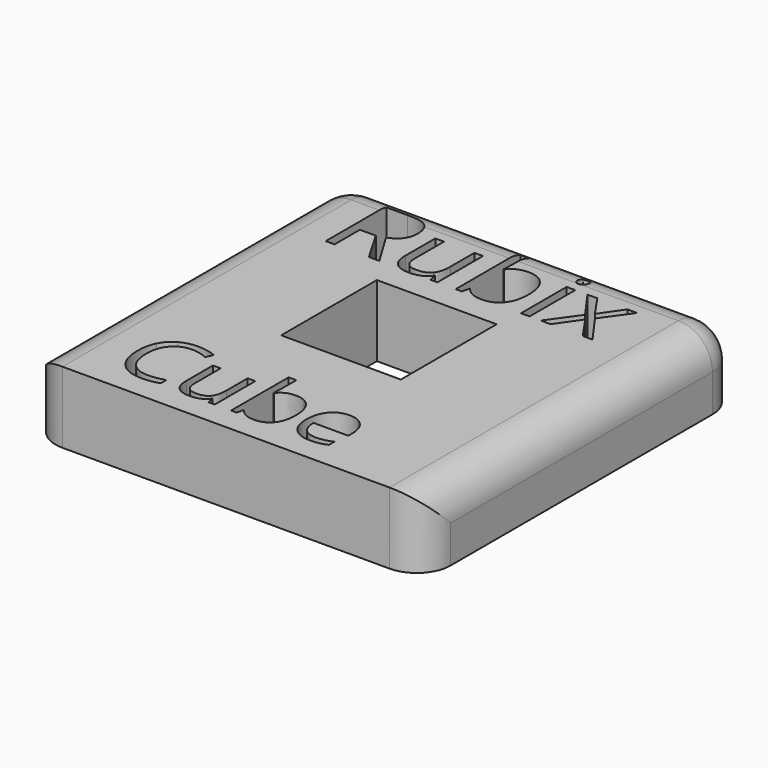
from build123d import *

# Parameters (mm, degrees)
F0_W         = 58.1
F0_H         = 58.1
F0_W_2       = 17.6
F0_H_2       = 17.6
F0_W_3       = 1.2705228995
F0_H_3       = 8.3844719282
F1_DEPTH     = 10.5
F2_T1_DEPTH  = 48.1
F2_T3_DEPTH  = 65.6
F2_T5_DEPTH  = 35.5
F2_T7_DEPTH  = 18
F2_S11_W     = 5
F2_S11_H     = 5
F2_T12_DEPTH = 5
F2_S17_W     = 5
F2_S17_H     = 5
F2_T18_DEPTH = 5


# Not quite as in the source:
# - a fillet or chamfer that OpenCascade refuses, or shapes differently, is made with other operations: its cross-section is extruded or revolved along the edge and cut away or added


with BuildPart() as f1:
    # F0 (on Top) → F1 (new body)
    with BuildSketch(Plane.XY):
        with Locations((-12.3929342572, -6.4361356199)):
            Rectangle(F0_W, F0_H)
        with BuildLine():
            add(Edge.make_bspline(
                [(-25.1530124377, -23.3911235684), (-26.2823661029, -22.8623510431), (-27.411719768, -22.8623510431)],
                knots=[0, 0, 0, 1, 1, 1], degree=2))
            add(Edge.make_bspline(
                [(-27.411719768, -22.8623510431), (-29.0502617908, -22.8623510431), (-29.9990059102, -23.9536243824)],
                knots=[0, 0, 0, 1, 1, 1], degree=2))
            add(Edge.make_bspline(
                [(-29.9990059102, -23.9536243824), (-30.9477500297, -25.0448977216), (-30.9477500297, -26.9423859605)],
                knots=[0, 0, 0, 1, 1, 1], degree=2))
            add(Edge.make_bspline(
                [(-30.9477500297, -26.9423859605), (-30.9477500297, -28.8920986463), (-30.0327341989, -29.957259762)],
                knots=[0, 0, 0, 1, 1, 1], degree=2))
            add(Edge.make_bspline(
                [(-30.0327341989, -29.957259762), (-29.1177183681, -31.0224208778), (-27.4247758797, -31.0224208778)],
                knots=[0, 0, 0, 1, 1, 1], degree=2))
            add(Edge.make_bspline(
                [(-27.4247758797, -31.0224208778), (-26.3846389781, -31.0224208778), (-25.0507395625, -30.6481456747)],
                knots=[0, 0, 0, 1, 1, 1], degree=2))
            Line((-25.0507395625, -30.6481456747), (-25.0507395625, -31.6599943342))
            add(Edge.make_bspline(
                [(-25.0507395625, -31.6599943342), (-26.0843484082, -32.0495016676), (-27.6010333881, -32.0495016676)],
                knots=[0, 0, 0, 1, 1, 1], degree=2))
            add(Edge.make_bspline(
                [(-27.6010333881, -32.0495016676), (-29.7966361783, -32.0495016676), (-30.9901823928, -30.715602252)],
                knots=[0, 0, 0, 1, 1, 1], degree=2))
            add(Edge.make_bspline(
                [(-30.9901823928, -30.715602252), (-32.1837286073, -29.3817028364), (-32.1837286073, -26.9271538301)],
                knots=[0, 0, 0, 1, 1, 1], degree=2))
            add(Edge.make_bspline(
                [(-32.1837286073, -26.9271538301), (-32.1837286073, -25.3908846826), (-31.6092596909, -24.235418794)],
                knots=[0, 0, 0, 1, 1, 1], degree=2))
            add(Edge.make_bspline(
                [(-31.6092596909, -24.235418794), (-31.0347907746, -23.0799529054), (-29.9500454912, -22.4543475514)],
                knots=[0, 0, 0, 1, 1, 1], degree=2))
            add(Edge.make_bspline(
                [(-29.9500454912, -22.4543475514), (-28.8653002079, -21.8287421974), (-27.3964876376, -21.8287421974)],
                knots=[0, 0, 0, 1, 1, 1], degree=2))
            add(Edge.make_bspline(
                [(-27.3964876376, -21.8287421974), (-25.8341062666, -21.8287421974), (-24.6634082477, -22.3988590765)],
                knots=[0, 0, 0, 1, 1, 1], degree=2))
            Line((-24.6634082477, -22.3988590765), (-25.1530124377, -23.3911235684))
        make_face(mode=Mode.SUBTRACT)
        with BuildLine():
            Line((-23.1314911374, -24.4595487121), (-21.9890813605, -24.4595487121))
            Line((-21.9890813605, -24.4595487121), (-21.9890813605, -29.2946620915))
            add(Edge.make_bspline(
                [(-21.9890813605, -29.2946620915), (-21.9890813605, -30.2064138943), (-21.5745498129, -30.6546737306)],
                knots=[0, 0, 0, 1, 1, 1], degree=2))
            add(Edge.make_bspline(
                [(-21.5745498129, -30.6546737306), (-21.1600182653, -31.1029335668), (-20.2765547046, -31.1029335668)],
                knots=[0, 0, 0, 1, 1, 1], degree=2))
            add(Edge.make_bspline(
                [(-20.2765547046, -31.1029335668), (-19.1058566856, -31.1029335668), (-18.5662040672, -30.4642721011)],
                knots=[0, 0, 0, 1, 1, 1], degree=2))
            add(Edge.make_bspline(
                [(-18.5662040672, -30.4642721011), (-18.0265514488, -29.8256106354), (-18.0265514488, -28.3763822327)],
                knots=[0, 0, 0, 1, 1, 1], degree=2))
            Line((-18.0265514488, -28.3763822327), (-18.0265514488, -24.4595487121))
            Line((-18.0265514488, -24.4595487121), (-16.8971977837, -24.4595487121))
            Line((-16.8971977837, -24.4595487121), (-16.8971977837, -31.9124124944))
            Line((-16.8971977837, -31.9124124944), (-17.8285337542, -31.9124124944))
            Line((-17.8285337542, -31.9124124944), (-17.9917351508, -30.9136199467))
            Line((-17.9917351508, -30.9136199467), (-18.0526636723, -30.9136199467))
            add(Edge.make_bspline(
                [(-18.0526636723, -30.9136199467), (-18.3986506333, -31.4641526582), (-19.0144639035, -31.7568271629)],
                knots=[0, 0, 0, 1, 1, 1], degree=2))
            add(Edge.make_bspline(
                [(-19.0144639035, -31.7568271629), (-19.6302771736, -32.0495016676), (-20.4201719336, -32.0495016676)],
                knots=[0, 0, 0, 1, 1, 1], degree=2))
            add(Edge.make_bspline(
                [(-20.4201719336, -32.0495016676), (-21.7801835727, -32.0495016676), (-22.4558373551, -31.4032241367)],
                knots=[0, 0, 0, 1, 1, 1], degree=2))
            add(Edge.make_bspline(
                [(-22.4558373551, -31.4032241367), (-23.1314911374, -30.7569466058), (-23.1314911374, -29.3360064453)],
                knots=[0, 0, 0, 1, 1, 1], degree=2))
            Line((-23.1314911374, -29.3360064453), (-23.1314911374, -24.4595487121))
        make_face(mode=Mode.SUBTRACT)
        with BuildLine():
            add(Edge.make_bspline(
                [(-13.3742236337, -25.451813204), (-12.5865048924, -24.3376916692), (-11.0350036145, -24.3376916692)],
                knots=[0, 0, 0, 1, 1, 1], degree=2))
            add(Edge.make_bspline(
                [(-11.0350036145, -24.3376916692), (-9.5661910442, -24.3376916692), (-8.7534480887, -25.3408362542)],
                knots=[0, 0, 0, 1, 1, 1], degree=2))
            add(Edge.make_bspline(
                [(-8.7534480887, -25.3408362542), (-7.9407051332, -26.3439808393), (-7.9407051332, -28.1783645381)],
                knots=[0, 0, 0, 1, 1, 1], degree=2))
            add(Edge.make_bspline(
                [(-7.9407051332, -28.1783645381), (-7.9407051332, -30.0149242555), (-8.7599761446, -31.0322129616)],
                knots=[0, 0, 0, 1, 1, 1], degree=2))
            add(Edge.make_bspline(
                [(-8.7599761446, -31.0322129616), (-9.579247156, -32.0495016676), (-11.0350036145, -32.0495016676)],
                knots=[0, 0, 0, 1, 1, 1], degree=2))
            add(Edge.make_bspline(
                [(-11.0350036145, -32.0495016676), (-11.763969853, -32.0495016676), (-12.3656390022, -31.7807633678)],
                knots=[0, 0, 0, 1, 1, 1], degree=2))
            add(Edge.make_bspline(
                [(-12.3656390022, -31.7807633678), (-12.9673081513, -31.5120250679), (-13.3742236337, -30.9527882819)],
                knots=[0, 0, 0, 1, 1, 1], degree=2))
            Line((-13.3742236337, -30.9527882819), (-13.4569123414, -30.9527882819))
            Line((-13.4569123414, -30.9527882819), (-13.6940983713, -31.9124124944))
            Line((-13.6940983713, -31.9124124944), (-14.5035772989, -31.9124124944))
            Line((-14.5035772989, -31.9124124944), (-14.5035772989, -21.3304339328))
            Line((-14.5035772989, -21.3304339328), (-13.3742236337, -21.3304339328))
            Line((-13.3742236337, -21.3304339328), (-13.3742236337, -23.9024879447))
            add(Edge.make_bspline(
                [(-13.3742236337, -23.9024879447), (-13.3742236337, -24.7663673379), (-13.4286240993, -25.451813204)],
                knots=[0, 0, 0, 1, 1, 1], degree=2))
            Line((-13.4286240993, -25.451813204), (-13.3742236337, -25.451813204))
        make_face(mode=Mode.SUBTRACT)
        with BuildLine():
            add(Edge.make_bspline(
                [(-1.5323302897, -31.9363486993), (-2.0654548522, -32.0495016676), (-2.8205333143, -32.0495016676)],
                knots=[0, 0, 0, 1, 1, 1], degree=2))
            add(Edge.make_bspline(
                [(-2.8205333143, -32.0495016676), (-4.4721314488, -32.0495016676), (-5.4284916334, -31.0420050454)],
                knots=[0, 0, 0, 1, 1, 1], degree=2))
            add(Edge.make_bspline(
                [(-5.4284916334, -31.0420050454), (-6.384851818, -30.0345084231), (-6.384851818, -28.247997134)],
                knots=[0, 0, 0, 1, 1, 1], degree=2))
            add(Edge.make_bspline(
                [(-6.384851818, -28.247997134), (-6.384851818, -26.4440776959), (-5.49703622, -25.3832686174)],
                knots=[0, 0, 0, 1, 1, 1], degree=2))
            add(Edge.make_bspline(
                [(-5.49703622, -25.3832686174), (-4.609220622, -24.3224595389), (-3.1121198097, -24.3224595389)],
                knots=[0, 0, 0, 1, 1, 1], degree=2))
            add(Edge.make_bspline(
                [(-3.1121198097, -24.3224595389), (-1.7129398354, -24.3224595389), (-0.8969328519, -25.2440034255)],
                knots=[0, 0, 0, 1, 1, 1], degree=2))
            add(Edge.make_bspline(
                [(-0.8969328519, -25.2440034255), (-0.0809258684, -26.1655473122), (-0.0809258684, -27.6757042363)],
                knots=[0, 0, 0, 1, 1, 1], degree=2))
            Line((-0.0809258684, -27.6757042363), (-0.0809258684, -28.3894383445))
            Line((-0.0809258684, -28.3894383445), (-5.2141537991, -28.3894383445))
            add(Edge.make_bspline(
                [(-5.2141537991, -28.3894383445), (-5.1793375011, -29.7015775739), (-4.5504681192, -30.3815833934)],
                knots=[0, 0, 0, 1, 1, 1], degree=2))
            add(Edge.make_bspline(
                [(-4.5504681192, -30.3815833934), (-3.9215987373, -31.061589213), (-2.7791889604, -31.061589213)],
                knots=[0, 0, 0, 1, 1, 1], degree=2))
            add(Edge.make_bspline(
                [(-2.7791889604, -31.061589213), (-1.5758506621, -31.061589213), (-0.400800606, -30.5589289112)],
                knots=[0, 0, 0, 1, 1, 1], degree=2))
            Line((-0.400800606, -30.5589289112), (-0.400800606, -31.5664255334))
            add(Edge.make_bspline(
                [(-0.400800606, -31.5664255334), (-0.9992057272, -31.8231957309), (-1.5323302897, -31.9363486993)],
                knots=[0, 0, 0, 1, 1, 1], degree=2))
        make_face(mode=Mode.SUBTRACT)
        with Locations((-12.8948209353, -4.9118663196)):
            Rectangle(F0_W_2, F0_H_2, mode=Mode.SUBTRACT)
        with BuildLine():
            Line((-28.6974735783, 12.4294076264), (-31.0328856132, 12.4294076264))
            Line((-31.0328856132, 12.4294076264), (-31.0328856132, 7.7781677246))
            Line((-31.0328856132, 7.7781677246), (-32.3327847646, 7.7781677246))
            Line((-32.3327847646, 7.7781677246), (-32.3327847646, 18.9631756778))
            Line((-32.3327847646, 18.9631756778), (-29.2654144505, 18.9631756778))
            add(Edge.make_bspline(
                [(-29.2654144505, 18.9631756778), (-27.2066287887, 18.9631756778), (-26.2237483568, 18.1749129155)],
                knots=[0, 0, 0, 1, 1, 1], degree=2))
            add(Edge.make_bspline(
                [(-26.2237483568, 18.1749129155), (-25.240867925, 17.3866501532), (-25.240867925, 15.8027805656)],
                knots=[0, 0, 0, 1, 1, 1], degree=2))
            add(Edge.make_bspline(
                [(-25.240867925, 15.8027805656), (-25.240867925, 13.5848735388), (-27.4905992248, 12.8039548395)],
                knots=[0, 0, 0, 1, 1, 1], degree=2))
            Line((-27.4905992248, 12.8039548395), (-24.4526051627, 7.7781677246))
            Line((-24.4526051627, 7.7781677246), (-25.9899623513, 7.7781677246))
            Line((-25.9899623513, 7.7781677246), (-28.6974735783, 12.4294076264))
        make_face(mode=Mode.SUBTRACT)
        with BuildLine():
            Line((-22.9299361001, 16.1626396528), (-21.6447250746, 16.1626396528))
            Line((-21.6447250746, 16.1626396528), (-21.6447250746, 10.7231369887))
            add(Edge.make_bspline(
                [(-21.6447250746, 10.7231369887), (-21.6447250746, 9.6974161893), (-21.1783770739, 9.1931238631)],
                knots=[0, 0, 0, 1, 1, 1], degree=2))
            add(Edge.make_bspline(
                [(-21.1783770739, 9.1931238631), (-20.7120290733, 8.688831537), (-19.7181325469, 8.688831537)],
                knots=[0, 0, 0, 1, 1, 1], degree=2))
            add(Edge.make_bspline(
                [(-19.7181325469, 8.688831537), (-18.4010972484, 8.688831537), (-17.7939880402, 9.4073257007)],
                knots=[0, 0, 0, 1, 1, 1], degree=2))
            add(Edge.make_bspline(
                [(-17.7939880402, 9.4073257007), (-17.1868788319, 10.1258198645), (-17.1868788319, 11.7562018511)],
                knots=[0, 0, 0, 1, 1, 1], degree=2))
            Line((-17.1868788319, 11.7562018511), (-17.1868788319, 16.1626396528))
            Line((-17.1868788319, 16.1626396528), (-15.9163559325, 16.1626396528))
            Line((-15.9163559325, 16.1626396528), (-15.9163559325, 7.7781677246))
            Line((-15.9163559325, 7.7781677246), (-16.9641089209, 7.7781677246))
            Line((-16.9641089209, 7.7781677246), (-17.1477104959, 8.901809364))
            Line((-17.1477104959, 8.901809364), (-17.2162550839, 8.901809364))
            add(Edge.make_bspline(
                [(-17.2162550839, 8.901809364), (-17.6054904231, 8.2824600508), (-18.2982803664, 7.9532012262)],
                knots=[0, 0, 0, 1, 1, 1], degree=2))
            add(Edge.make_bspline(
                [(-18.2982803664, 7.9532012262), (-18.9910703096, 7.6239424016), (-19.879701933, 7.6239424016)],
                knots=[0, 0, 0, 1, 1, 1], degree=2))
            add(Edge.make_bspline(
                [(-19.879701933, 7.6239424016), (-21.4097150585, 7.6239424016), (-22.1698255793, 8.3510046388)],
                knots=[0, 0, 0, 1, 1, 1], degree=2))
            add(Edge.make_bspline(
                [(-22.1698255793, 8.3510046388), (-22.9299361001, 9.0780668761), (-22.9299361001, 10.6766245897)],
                knots=[0, 0, 0, 1, 1, 1], degree=2))
            Line((-22.9299361001, 10.6766245897), (-22.9299361001, 16.1626396528))
        make_face(mode=Mode.SUBTRACT)
        with BuildLine():
            add(Edge.make_bspline(
                [(-11.953009932, 15.0463420764), (-11.0668263296, 16.2997288288), (-9.321387356, 16.2997288288)],
                knots=[0, 0, 0, 1, 1, 1], degree=2))
            add(Edge.make_bspline(
                [(-9.321387356, 16.2997288288), (-7.6689731803, 16.2997288288), (-6.7546373365, 15.1711911474)],
                knots=[0, 0, 0, 1, 1, 1], degree=2))
            add(Edge.make_bspline(
                [(-6.7546373365, 15.1711911474), (-5.8403014927, 14.042653466), (-5.8403014927, 11.9789717622)],
                knots=[0, 0, 0, 1, 1, 1], degree=2))
            add(Edge.make_bspline(
                [(-5.8403014927, 11.9789717622), (-5.8403014927, 9.9128420374), (-6.7619813995, 8.7683922195)],
                knots=[0, 0, 0, 1, 1, 1], degree=2))
            add(Edge.make_bspline(
                [(-6.7619813995, 8.7683922195), (-7.6836613063, 7.6239424016), (-9.321387356, 7.6239424016)],
                knots=[0, 0, 0, 1, 1, 1], degree=2))
            add(Edge.make_bspline(
                [(-9.321387356, 7.6239424016), (-10.1414743913, 7.6239424016), (-10.818352198, 7.9262729952)],
                knots=[0, 0, 0, 1, 1, 1], degree=2))
            add(Edge.make_bspline(
                [(-10.818352198, 7.9262729952), (-11.4952300048, 8.2286035888), (-11.953009932, 8.857744986)],
                knots=[0, 0, 0, 1, 1, 1], degree=2))
            Line((-11.953009932, 8.857744986), (-12.04603473, 8.857744986))
            Line((-12.04603473, 8.857744986), (-12.3128690191, 7.7781677246))
            Line((-12.3128690191, 7.7781677246), (-13.2235328314, 7.7781677246))
            Line((-13.2235328314, 7.7781677246), (-13.2235328314, 19.6828938521))
            Line((-13.2235328314, 19.6828938521), (-11.953009932, 19.6828938521))
            Line((-11.953009932, 19.6828938521), (-11.953009932, 16.789333029))
            add(Edge.make_bspline(
                [(-11.953009932, 16.789333029), (-11.953009932, 15.8174686916), (-12.014210457, 15.0463420764)],
                knots=[0, 0, 0, 1, 1, 1], degree=2))
            Line((-12.014210457, 15.0463420764), (-11.953009932, 15.0463420764))
        make_face(mode=Mode.SUBTRACT)
        with Locations((-2.9871330161, 11.9704036887)):
            Rectangle(F0_W_3, F0_H_3, mode=Mode.SUBTRACT)
        with BuildLine():
            add(Edge.make_bspline(
                [(-3.5159055523, 17.7954696604), (-3.7301073899, 18.0059994665), (-3.7301073899, 18.4344031416)],
                knots=[0, 0, 0, 1, 1, 1], degree=2))
            add(Edge.make_bspline(
                [(-3.7301073899, 18.4344031416), (-3.7301073899, 18.8701508798), (-3.5159055523, 19.0733366229)],
                knots=[0, 0, 0, 1, 1, 1], degree=2))
            add(Edge.make_bspline(
                [(-3.5159055523, 19.0733366229), (-3.3017037147, 19.2765223659), (-2.9785649426, 19.2765223659)],
                knots=[0, 0, 0, 1, 1, 1], degree=2))
            add(Edge.make_bspline(
                [(-2.9785649426, 19.2765223659), (-2.6725623175, 19.2765223659), (-2.4510164169, 19.0696645914)],
                knots=[0, 0, 0, 1, 1, 1], degree=2))
            add(Edge.make_bspline(
                [(-2.4510164169, 19.0696645914), (-2.2294705163, 18.8628068168), (-2.2294705163, 18.4344031416)],
                knots=[0, 0, 0, 1, 1, 1], degree=2))
            add(Edge.make_bspline(
                [(-2.2294705163, 18.4344031416), (-2.2294705163, 18.0059994665), (-2.4510164169, 17.7954696604)],
                knots=[0, 0, 0, 1, 1, 1], degree=2))
            add(Edge.make_bspline(
                [(-2.4510164169, 17.7954696604), (-2.6725623175, 17.5849398543), (-2.9785649426, 17.5849398543)],
                knots=[0, 0, 0, 1, 1, 1], degree=2))
            add(Edge.make_bspline(
                [(-2.9785649426, 17.5849398543), (-3.3017037147, 17.5849398543), (-3.5159055523, 17.7954696604)],
                knots=[0, 0, 0, 1, 1, 1], degree=2))
        make_face(mode=Mode.SUBTRACT)
        Polygon((-0.7068014537, 7.7781677246), (2.3605688604, 12.0695485392), (-0.5550241517, 16.1626396528), (0.8917562599, 16.1626396528), (3.1023192237, 12.9508360996), (5.3055381246, 16.1626396528), (6.7376304101, 16.1626396528), (3.822037398, 12.0695485392), (6.8894077122, 7.7781677246), (5.4524193846, 7.7781677246), (3.1023192237, 11.1760208739), (0.7301868738, 7.7781677246), align=None, mode=Mode.SUBTRACT)
    extrude(amount=F1_DEPTH)

    # F2: fillet of radius 5 on 7 edges, made by hand

    # F2_s2 → F2_t1 (cut)
    with BuildSketch(Plane.YZ.offset(-36.4429342572)):
        with BuildLine():
            ThreePointArc((22.6138643801, 5.5), (21.1493982861, 9.0355339059), (17.6138643801, 10.5))
            Line((17.6138643801, 10.5), (22.6138643801, 10.5))
            Line((22.6138643801, 10.5), (22.6138643801, 5.5))
        make_face()
    extrude(amount=F2_T1_DEPTH, mode=Mode.SUBTRACT)

    # F2_s4 → F2_t3 (cut)
    with BuildSketch(Plane.XZ.offset(-17.6138643801)):
        with BuildLine():
            ThreePointArc((16.6570657428, 5.5), (15.1925996488, 9.0355339059), (11.6570657428, 10.5))
            Line((11.6570657428, 10.5), (16.6570657428, 10.5))
            Line((16.6570657428, 10.5), (16.6570657428, 5.5))
        make_face()
        with BuildLine():
            ThreePointArc((-41.4429342572, 5.5), (-39.9784681631, 9.0355339059), (-36.4429342572, 10.5))
            Line((-36.4429342572, 10.5), (-41.4429342572, 10.5))
            Line((-41.4429342572, 10.5), (-41.4429342572, 5.5))
        make_face()
    extrude(amount=F2_T3_DEPTH, mode=Mode.SUBTRACT)

    # F2_s6 → F2_t5 (cut)
    with BuildSketch(Plane.XY.offset(-12.5)):
        with BuildLine():
            ThreePointArc((11.6570657428, -35.4861356199), (15.1925996488, -34.0216695258), (16.6570657428, -30.4861356199))
            Line((16.6570657428, -30.4861356199), (16.6570657428, -35.4861356199))
            Line((16.6570657428, -35.4861356199), (11.6570657428, -35.4861356199))
        make_face()
        with BuildLine():
            ThreePointArc((-41.4429342572, -30.4861356199), (-39.9784681631, -34.0216695258), (-36.4429342572, -35.4861356199))
            Line((-36.4429342572, -35.4861356199), (-41.4429342572, -35.4861356199))
            Line((-41.4429342572, -35.4861356199), (-41.4429342572, -30.4861356199))
        make_face()
    extrude(amount=F2_T5_DEPTH, mode=Mode.SUBTRACT)

    # F2_s8 → F2_t7 (cut)
    with BuildSketch(Plane.XY.offset(-12.5)):
        with BuildLine():
            ThreePointArc((11.6570657428, 22.6138643801), (15.1925996488, 21.1493982861), (16.6570657428, 17.6138643801))
            Line((16.6570657428, 17.6138643801), (16.6570657428, 22.6138643801))
            Line((16.6570657428, 22.6138643801), (11.6570657428, 22.6138643801))
        make_face()
        with BuildLine():
            ThreePointArc((-36.4429342572, 22.6138643801), (-39.9784681631, 21.1493982861), (-41.4429342572, 17.6138643801))
            Line((-41.4429342572, 17.6138643801), (-41.4429342572, 22.6138643801))
            Line((-41.4429342572, 22.6138643801), (-36.4429342572, 22.6138643801))
        make_face()
    extrude(amount=F2_T7_DEPTH, mode=Mode.SUBTRACT)


with BuildPart() as f2_tool10:
    # F2_s11 → F2_t12 (new body)
    with BuildSketch(Plane.XZ.offset(-17.6138643801)):
        with Locations((14.1570657428, 8)):
            Rectangle(F2_S11_W, F2_S11_H)
    extrude(amount=-F2_T12_DEPTH)

    # F2_s13 → F2_t14 (revolve, cut)
    with BuildSketch(Plane(origin=(11.6570657428, 17.6138643801, 5.5), x_dir=(-0.7071067812, 0, -0.7071067812), z_dir=(0.7071067812, 0, -0.7071067812))):
        with BuildLine():
            ThreePointArc((0, -5), (5, 0), (0, 5))
            Line((0, 5), (0, -5))
        make_face()
    revolve(axis=Axis((11.6570657428, 17.6138643801, 5.5), (0, 1, 0)), mode=Mode.SUBTRACT)


with BuildPart() as f1_1:
    add(f1.part)

    # F2_t9: cut F2_tool10
    add(f2_tool10.part, mode=Mode.SUBTRACT)


with BuildPart() as f2_tool16:
    # F2_s17 → F2_t18 (new body)
    with BuildSketch(Plane.XZ.offset(-17.6138643801)):
        with Locations((-38.9429342572, 8)):
            Rectangle(F2_S17_W, F2_S17_H)
    extrude(amount=-F2_T18_DEPTH)

    # F2_s19 → F2_t20 (revolve, cut)
    with BuildSketch(Plane(origin=(-36.4429342572, 17.6138643801, 5.5), x_dir=(0.7071067812, 0, -0.7071067812), z_dir=(0.7071067812, 0, 0.7071067812))):
        with BuildLine():
            ThreePointArc((0, -5), (5, 0), (0, 5))
            Line((0, 5), (0, -5))
        make_face()
    revolve(axis=Axis((-36.4429342572, 17.6138643801, 5.5), (0, 1, 0)), mode=Mode.SUBTRACT)


with BuildPart() as f1_2:
    add(f1_1.part)

    # F2_t15: cut F2_tool16
    add(f2_tool16.part, mode=Mode.SUBTRACT)


solid = f1_2.part
